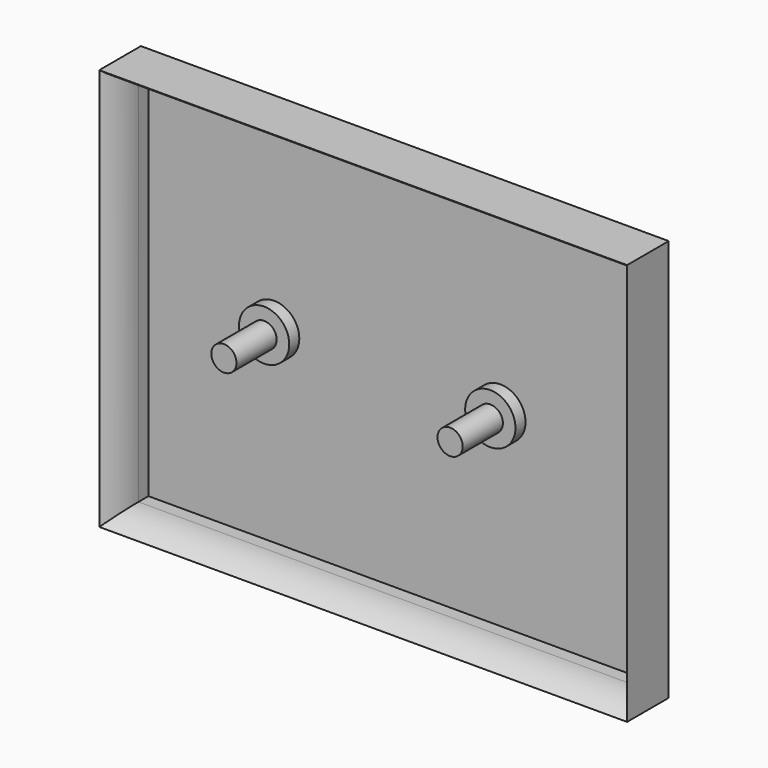
from build123d import *

# Parameters (mm, degrees)
F0_W         = 133.35
F0_H         = 101.6
F1_DEPTH     = 19.05
F2_T         = -3.175
F3_R         = 6.35
F4_DEPTH     = 3.175
F5_R         = 3.175
F6_DEPTH     = 12.7
F7_R         = 3.175
F8_DEPTH     = 12.7
F9_T1_DEPTH  = 95.25
F9_T3_DEPTH  = 127
F9_T9_DEPTH  = 158.75
F9_T15_DEPTH = 127
F9_T24_DEPTH = 158.75
F9_T30_DEPTH = 127
F9_T39_DEPTH = 127
F9_T45_DEPTH = 158.75
F9_T54_DEPTH = 158.75
F9_T60_DEPTH = 127
F10_SIZE     = 1.6002


# Not quite as in the source:
# - a fillet or chamfer that OpenCascade refuses, or shapes differently, is made with other operations: its cross-section is extruded or revolved along the edge and cut away or added


with BuildPart() as f1:
    # F0 (on Front) → F1 (new body)
    with BuildSketch(Plane.XZ):
        with Locations((-34.2663429767, 0.1884810627)):
            Rectangle(F0_W, F0_H)
    extrude(amount=F1_DEPTH)

    # F2
    f2_openings = [f1.faces().sort_by_distance(p)[0] for p in [
        (-34.266343, -19.05, 0.188481),
    ]]
    offset(amount=F2_T, openings=f2_openings)

    # F3 (on face) → F4 (join)
    with BuildSketch(Plane.XZ.offset(3.175)):
        with Locations((-66.0163429767, 0)):
            Circle(F3_R)
        with Locations((-8.8663429767, 0)):
            Circle(F3_R)
    extrude(amount=F4_DEPTH)

    # F5 (on face) → F6 (join)
    with BuildSketch(Plane.XZ.offset(6.35)):
        with Locations((-66.0163429767, 0)):
            Circle(F5_R)
    extrude(amount=F6_DEPTH)

    # F7 (on face) → F8 (join)
    with BuildSketch(Plane.XZ.offset(6.35)):
        with Locations((-8.8663429767, 0)):
            Circle(F7_R)
    extrude(amount=F8_DEPTH)

    # F9: fillet of radius 12.7 on 4 edges, made by hand

    # F9_s2 → F9_t1 (cut)
    with BuildSketch(Plane.XY.offset(-47.4365189373)):
        with BuildLine():
            ThreePointArc((-110.4663429767, -19.05), (-101.4860868556, -15.3302561211), (-97.7663429767, -6.35))
            Line((-97.7663429767, -6.35), (-97.7663429767, -19.05))
            Line((-97.7663429767, -19.05), (-110.4663429767, -19.05))
        make_face()
        with BuildLine():
            ThreePointArc((41.9336570233, -19.05), (32.9534009023, -15.3302561211), (29.2336570233, -6.35))
            Line((29.2336570233, -6.35), (29.2336570233, -19.05))
            Line((29.2336570233, -19.05), (41.9336570233, -19.05))
        make_face()
    extrude(amount=F9_T1_DEPTH, mode=Mode.SUBTRACT)

    # F9_s4 → F9_t3 (cut)
    with BuildSketch(Plane.YZ.offset(-97.7663429767)):
        with BuildLine():
            ThreePointArc((-19.05, -60.1365189373), (-15.3302561211, -51.1562628163), (-6.35, -47.4365189373))
            Line((-6.35, -47.4365189373), (-19.05, -47.4365189373))
            Line((-19.05, -47.4365189373), (-19.05, -60.1365189373))
        make_face()
        with BuildLine():
            ThreePointArc((-19.05, 60.5134810627), (-15.3302561211, 51.5332249416), (-6.35, 47.8134810627))
            Line((-6.35, 47.8134810627), (-19.05, 47.8134810627))
            Line((-19.05, 47.8134810627), (-19.05, 60.5134810627))
        make_face()
    extrude(amount=F9_T3_DEPTH, mode=Mode.SUBTRACT)


with BuildPart() as f9_tool7:
    # F9_s8 → F9_t9 (new body)
    with BuildSketch(Plane.YZ.offset(29.2336570233)):
        with BuildLine():
            ThreePointArc((-19.05, 60.5134810627), (-15.3302561211, 51.5332249416), (-6.35, 47.8134810627))
            Line((-6.35, 47.8134810627), (-19.05, 47.8134810627))
            Line((-19.05, 47.8134810627), (-19.05, 60.5134810627))
        make_face()
    extrude(amount=-F9_T9_DEPTH)

    split(bisect_by=Plane.XY.offset(50.9884810627), keep=Keep.BOTTOM)

    split(bisect_by=Plane.YZ.offset(-100.9413429767), keep=Keep.TOP)

    split(bisect_by=Plane.YZ.offset(-97.7663429767), keep=Keep.BOTTOM)


with BuildPart() as f9_tool13:
    # F9_s14 → F9_t15 (new body)
    with BuildSketch(Plane.XY.offset(79.5634810627)):
        with BuildLine():
            ThreePointArc((-110.4663429767, -19.05), (-101.4860868556, -15.3302561211), (-97.7663429767, -6.35))
            Line((-97.7663429767, -6.35), (-97.7663429767, -19.05))
            Line((-97.7663429767, -19.05), (-110.4663429767, -19.05))
        make_face()
    extrude(amount=-F9_T15_DEPTH)

    split(bisect_by=Plane.XY.offset(50.9884810627), keep=Keep.BOTTOM)

    split(bisect_by=Plane.YZ.offset(-100.9413429767), keep=Keep.TOP)

    split(bisect_by=Plane.XY.offset(47.8134810627), keep=Keep.TOP)


with BuildPart() as f9_tool7_1:
    add(f9_tool7.part)

    # F9_t19: intersect F9_tool13
    add(f9_tool13.part, mode=Mode.INTERSECT)


with BuildPart() as f1_1:
    add(f1.part)

    # F9_t5: cut F9_tool7
    add(f9_tool7_1.part, mode=Mode.SUBTRACT)


with BuildPart() as f9_tool22:
    # F9_s23 → F9_t24 (new body)
    with BuildSketch(Plane.YZ.offset(-129.5163429767)):
        with BuildLine():
            ThreePointArc((-19.05, -60.1365189373), (-15.3302561211, -51.1562628163), (-6.35, -47.4365189373))
            Line((-6.35, -47.4365189373), (-19.05, -47.4365189373))
            Line((-19.05, -47.4365189373), (-19.05, -60.1365189373))
        make_face()
    extrude(amount=F9_T24_DEPTH)

    split(bisect_by=Plane.YZ.offset(-100.9413429767), keep=Keep.TOP)

    split(bisect_by=Plane.XY.offset(-50.6115189373), keep=Keep.TOP)

    split(bisect_by=Plane.YZ.offset(-97.7663429767), keep=Keep.BOTTOM)


with BuildPart() as f9_tool28:
    # F9_s29 → F9_t30 (new body)
    with BuildSketch(Plane.XY.offset(47.8134810627)):
        with BuildLine():
            ThreePointArc((-110.4663429767, -19.05), (-101.4860868556, -15.3302561211), (-97.7663429767, -6.35))
            Line((-97.7663429767, -6.35), (-97.7663429767, -19.05))
            Line((-97.7663429767, -19.05), (-110.4663429767, -19.05))
        make_face()
    extrude(amount=-F9_T30_DEPTH)

    split(bisect_by=Plane.YZ.offset(-100.9413429767), keep=Keep.TOP)

    split(bisect_by=Plane.XY.offset(-50.6115189373), keep=Keep.TOP)

    split(bisect_by=Plane.XY.offset(-47.4365189373), keep=Keep.BOTTOM)


with BuildPart() as f9_tool22_1:
    add(f9_tool22.part)

    # F9_t34: intersect F9_tool28
    add(f9_tool28.part, mode=Mode.INTERSECT)


with BuildPart() as f1_2:
    add(f1_1.part)

    # F9_t20: cut F9_tool22
    add(f9_tool22_1.part, mode=Mode.SUBTRACT)


with BuildPart() as f9_tool37:
    # F9_s38 → F9_t39 (new body)
    with BuildSketch(Plane.XY.offset(-79.1865189373)):
        with BuildLine():
            ThreePointArc((41.9336570233, -19.05), (32.9534009023, -15.3302561211), (29.2336570233, -6.35))
            Line((29.2336570233, -6.35), (29.2336570233, -19.05))
            Line((29.2336570233, -19.05), (41.9336570233, -19.05))
        make_face()
    extrude(amount=F9_T39_DEPTH)

    split(bisect_by=Plane.YZ.offset(32.4086570233), keep=Keep.BOTTOM)

    split(bisect_by=Plane.XY.offset(-50.6115189373), keep=Keep.TOP)

    split(bisect_by=Plane.XY.offset(-47.4365189373), keep=Keep.BOTTOM)


with BuildPart() as f9_tool43:
    # F9_s44 → F9_t45 (new body)
    with BuildSketch(Plane.YZ.offset(-97.7663429767)):
        with BuildLine():
            ThreePointArc((-19.05, -60.1365189373), (-15.3302561211, -51.1562628163), (-6.35, -47.4365189373))
            Line((-6.35, -47.4365189373), (-19.05, -47.4365189373))
            Line((-19.05, -47.4365189373), (-19.05, -60.1365189373))
        make_face()
    extrude(amount=F9_T45_DEPTH)

    split(bisect_by=Plane.YZ.offset(32.4086570233), keep=Keep.BOTTOM)

    split(bisect_by=Plane.XY.offset(-50.6115189373), keep=Keep.TOP)

    split(bisect_by=Plane.YZ.offset(29.2336570233), keep=Keep.TOP)


with BuildPart() as f9_tool37_1:
    add(f9_tool37.part)

    # F9_t49: intersect F9_tool43
    add(f9_tool43.part, mode=Mode.INTERSECT)


with BuildPart() as f1_3:
    add(f1_2.part)

    # F9_t35: cut F9_tool37
    add(f9_tool37_1.part, mode=Mode.SUBTRACT)


with BuildPart() as f9_tool52:
    # F9_s53 → F9_t54 (new body)
    with BuildSketch(Plane.YZ.offset(60.9836570233)):
        with BuildLine():
            ThreePointArc((-19.05, 60.5134810627), (-15.3302561211, 51.5332249416), (-6.35, 47.8134810627))
            Line((-6.35, 47.8134810627), (-19.05, 47.8134810627))
            Line((-19.05, 47.8134810627), (-19.05, 60.5134810627))
        make_face()
    extrude(amount=-F9_T54_DEPTH)

    split(bisect_by=Plane.XY.offset(50.9884810627), keep=Keep.BOTTOM)

    split(bisect_by=Plane.YZ.offset(32.4086570233), keep=Keep.BOTTOM)

    split(bisect_by=Plane.YZ.offset(29.2336570233), keep=Keep.TOP)


with BuildPart() as f9_tool58:
    # F9_s59 → F9_t60 (new body)
    with BuildSketch(Plane.XY.offset(-47.4365189373)):
        with BuildLine():
            ThreePointArc((41.9336570233, -19.05), (32.9534009023, -15.3302561211), (29.2336570233, -6.35))
            Line((29.2336570233, -6.35), (29.2336570233, -19.05))
            Line((29.2336570233, -19.05), (41.9336570233, -19.05))
        make_face()
    extrude(amount=F9_T60_DEPTH)

    split(bisect_by=Plane.XY.offset(50.9884810627), keep=Keep.BOTTOM)

    split(bisect_by=Plane.YZ.offset(32.4086570233), keep=Keep.BOTTOM)

    split(bisect_by=Plane.XY.offset(47.8134810627), keep=Keep.TOP)


with BuildPart() as f9_tool52_1:
    add(f9_tool52.part)

    # F9_t64: intersect F9_tool58
    add(f9_tool58.part, mode=Mode.INTERSECT)


with BuildPart() as f1_4:
    add(f1_3.part)

    # F9_t50: cut F9_tool52
    add(f9_tool52_1.part, mode=Mode.SUBTRACT)

    # F10
    f10_edges = [f1_4.edges().sort_by_distance(p)[0] for p in [
        (-34.266343, 0, 50.988481),
        (-100.941343, 0, 0.188481),
        (-34.266343, 0, -50.611519),
        (32.408657, 0, 0.188481),
    ]]
    chamfer(f10_edges, length=F10_SIZE)


solid = f1_4.part
